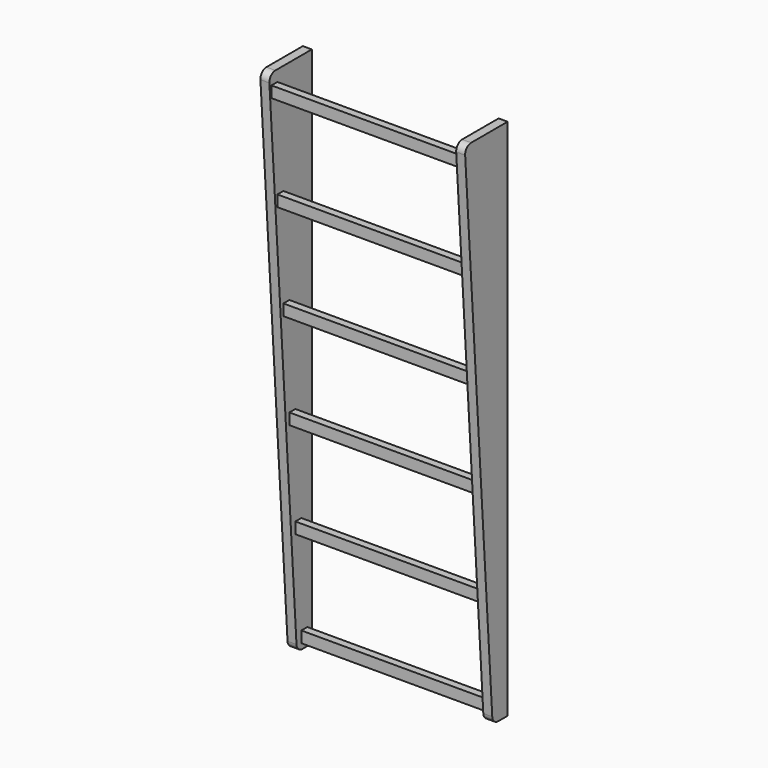
from build123d import *

# Parameters (mm, degrees)
F0_W          = 24
F0_H          = 150
F1_DEPTH      = 1400
F2_W          = 20
F2_H          = 30
F3_DEPTH      = 500
F4_T1_DEPTH   = 7823.3610770598
F4_2_T1_DEPTH = 7823.3610770598
F12_R         = 20
F12_2_R       = 20


# Not quite as in the source:
# - a fillet or chamfer that OpenCascade refuses, or shapes differently, is made with other operations: its cross-section is extruded or revolved along the edge and cut away or added
# - two fillets or chamfers of one size are made in one step


with BuildPart() as f1:
    # F0 (on Top) → F1 (new body)
    with BuildSketch(Plane.XY):
        with Locations((-262, 0)):
            Rectangle(F0_W, F0_H)
    extrude(amount=F1_DEPTH)

    # F4: chamfer of 100 x 1500 on 1 edges, made by hand

    # F4_s2 → F4_t1 (cut)
    with BuildSketch(Plane.YZ.offset(-4173.6805385299)):
        Polygon((-75, 1500), (25, 0), (-75, 0), align=None)
    extrude(amount=F4_T1_DEPTH, mode=Mode.SUBTRACT)

    # F12
    f12_edges = [f1.edges().sort_by_distance(p)[0] for p in [
        (-262, -68.333333, 1400),
        (-262, 25, 0),
    ]]
    fillet(f12_edges, radius=F12_R)


with BuildPart() as f1b:
    # F0 (on Top) → F1, piece 2 (new body)
    with BuildSketch(Plane.XY):
        with Locations((262, 0)):
            Rectangle(F0_W, F0_H)
    extrude(amount=F1_DEPTH)

    # F4#2: chamfer of 100 x 1500 on 1 edges, made by hand

    # F4_2_s2 → F4_2_t1 (cut)
    with BuildSketch(Plane.YZ.offset(-3649.6805385299)):
        Polygon((-75, 1500), (25, 0), (-75, 0), align=None)
    extrude(amount=F4_2_T1_DEPTH, mode=Mode.SUBTRACT)

    # F12#2
    f12_2_edges = [f1b.edges().sort_by_distance(p)[0] for p in [
        (262, 25, 0),
        (262, -68.333333, 1400),
    ]]
    fillet(f12_2_edges, radius=F12_2_R)


with BuildPart() as f3:
    # F2 (on face) → F3 (new body, through all)
    with BuildSketch(Plane(origin=(250, 0, 0), x_dir=(0, -1, 0), z_dir=(-1, 0, 0))):
        with Locations((0, 1355)):
            Rectangle(F2_W, F2_H)
    extrude(amount=F3_DEPTH)


with BuildPart() as f3b:
    # F2 (on face) → F3, piece 2 (new body, through all)
    with BuildSketch(Plane(origin=(250, 0, 0), x_dir=(0, -1, 0), z_dir=(-1, 0, 0))):
        with Locations((0, 1090)):
            Rectangle(F2_W, F2_H)
    extrude(amount=F3_DEPTH)


with BuildPart() as f3c:
    # F2 (on face) → F3, piece 3 (new body, through all)
    with BuildSketch(Plane(origin=(250, 0, 0), x_dir=(0, -1, 0), z_dir=(-1, 0, 0))):
        with Locations((0, 825)):
            Rectangle(F2_W, F2_H)
    extrude(amount=F3_DEPTH)


with BuildPart() as f3d:
    # F2 (on face) → F3, piece 4 (new body, through all)
    with BuildSketch(Plane(origin=(250, 0, 0), x_dir=(0, -1, 0), z_dir=(-1, 0, 0))):
        with Locations((0, 560)):
            Rectangle(F2_W, F2_H)
    extrude(amount=F3_DEPTH)


with BuildPart() as f3e:
    # F2 (on face) → F3, piece 5 (new body, through all)
    with BuildSketch(Plane(origin=(250, 0, 0), x_dir=(0, -1, 0), z_dir=(-1, 0, 0))):
        with Locations((0, 30)):
            Rectangle(F2_W, F2_H)
    extrude(amount=F3_DEPTH)


with BuildPart() as f3f:
    # F2 (on face) → F3, piece 6 (new body, through all)
    with BuildSketch(Plane(origin=(250, 0, 0), x_dir=(0, -1, 0), z_dir=(-1, 0, 0))):
        with Locations((0, 295)):
            Rectangle(F2_W, F2_H)
    extrude(amount=F3_DEPTH)


with BuildPart() as f3_1:
    # F6: moved
    add(f3.part.moved(Location((0, -50, 0))))


with BuildPart() as f3b_1:
    # F7: moved
    add(f3b.part.moved(Location((0, -30, 0))))


with BuildPart() as f3c_1:
    # F8: moved
    add(f3c.part.moved(Location((0, -10, 0))))


with BuildPart() as f3d_1:
    # F9: moved
    add(f3d.part.moved(Location((0, 10, 0))))


with BuildPart() as f3f_1:
    # F10: moved
    add(f3f.part.moved(Location((0, 30, 0))))


with BuildPart() as f3e_1:
    # F11: moved
    add(f3e.part.moved(Location((0, 50, 0))))


solid = Compound([f1.part, f1b.part, f3_1.part, f3b_1.part, f3c_1.part, f3d_1.part, f3f_1.part, f3e_1.part])
